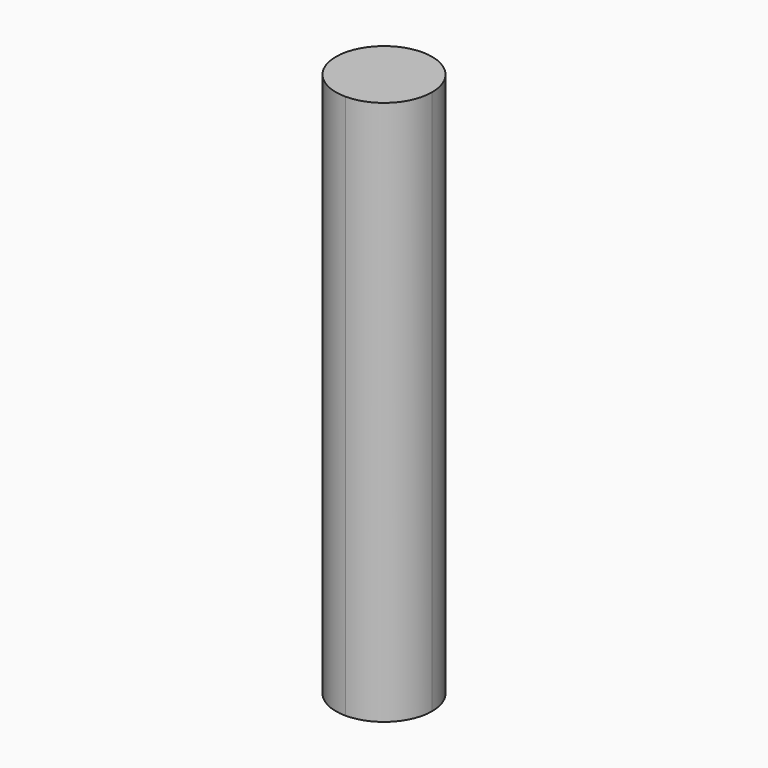
from build123d import *

# Parameters (mm, degrees)
F0_W          = 7.5
F0_H          = 35
F0_H_2        = 25
F1_DEPTH      = 7.5
F1_DEPTH_BACK = 7.5
F2_R          = 7.49999


# Not quite as in the source:
# - a fillet or chamfer is up to 0.001 mm smaller than in the source, because OpenCascade refuses the exact size


with BuildPart() as f1:
    # F0 (on Front) → F1 (new body, two sides)
    with BuildSketch(Plane.XZ) as f1_sk:
        Polygon((7.5, -12.5), (7.5, 12.5), (0, 12.5), (-7.5, 12.5), (-7.5, -12.5), align=None)
        with Locations((3.75, 30)):
            Rectangle(F0_W, F0_H)
        with Locations((-3.75, 60)):
            Rectangle(F0_W, F0_H_2)
        with Locations((3.75, 60)):
            Rectangle(F0_W, F0_H_2)
        with Locations((-3.75, 30)):
            Rectangle(F0_W, F0_H)
    extrude(amount=F1_DEPTH)
    extrude(f1_sk.sketch, amount=-F1_DEPTH_BACK)

    # F2 (radius 7.5 in the source; OpenCascade refuses exactly that, so slightly less here)
    f2_edges = [f1.edges().sort_by_distance(p)[0] for p in [
        (-7.5, -7.5, 30),
        (7.5, -7.5, 30),
        (-7.5, 7.5, 30),
        (7.5, 7.5, 30),
    ]]
    fillet(f2_edges, radius=F2_R)


solid = f1.part
